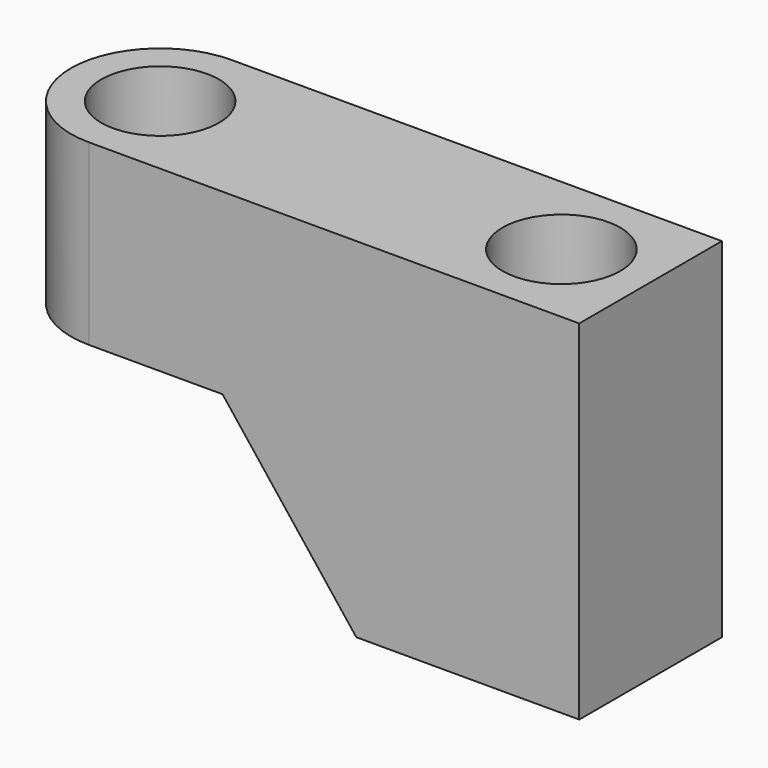
from build123d import *

# Parameters (mm, degrees)
F1_DEPTH       = 20
F2_R           = 9.99999
F4_D           = 13.2
F4_CBORE_D     = 19.25
F4_CBORE_DEPTH = 0


# Not quite as in the source:
# - a fillet or chamfer is up to 0.001 mm smaller than in the source, because OpenCascade refuses the exact size


with BuildPart() as f1:
    # F0 (on Front) → F1 (new body)
    with BuildSketch(Plane.XZ):
        Polygon((46.0956162758, 6.5648934066), (-18.9043837242, 6.5648934066), (-18.9043837242, -13.4351065934), (6.0956162758, -13.4351065934), (21.0956162758, -32.5433855138), (46.0956162758, -32.5433855138), align=None)
    extrude(amount=F1_DEPTH)

    # F2 (radius 10 in the source; OpenCascade refuses exactly that, so slightly less here)
    f2_edges = [f1.edges().sort_by_distance(p)[0] for p in [
        (-18.904384, 0, -3.435107),
        (-18.904384, -20, -3.435107),
    ]]
    fillet(f2_edges, radius=F2_R)

    # F4 (through all)
    with Locations(Plane.XY.offset(6.5648934066)):
        with Locations((-8.9043837242, -10), (36.0956162758, -10)):
            CounterBoreHole(F4_D / 2, F4_CBORE_D / 2, F4_CBORE_DEPTH)


solid = f1.part
